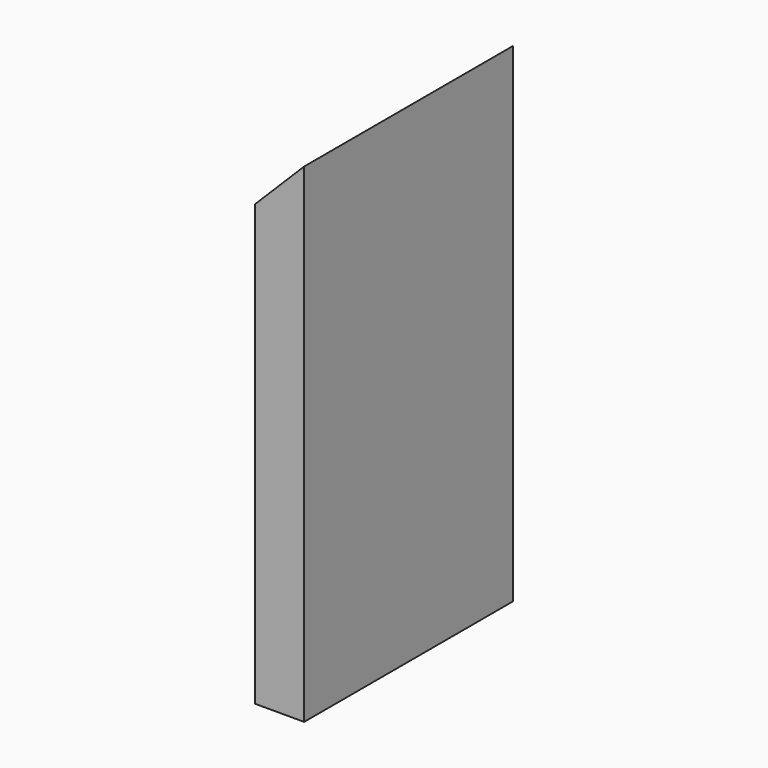
from build123d import *

# Parameters (mm, degrees)
F0_W     = 19.05
F0_H     = 101.6
F1_DEPTH = 190.5
F2_SIZE  = 19.04999


# Not quite as in the source:
# - a fillet or chamfer is up to 0.001 mm smaller than in the source, because OpenCascade refuses the exact size


with BuildPart() as f1:
    # F0 (on Top) → F1 (new body)
    with BuildSketch(Plane.XY):
        Rectangle(F0_W, F0_H)
    extrude(amount=F1_DEPTH)

    # F2 (size 19.05 in the source; OpenCascade refuses exactly that, so slightly less here)
    f2_edges = [f1.edges().sort_by_distance(p)[0] for p in [
        (-9.525, 0, 190.5),
    ]]
    chamfer(f2_edges, length=F2_SIZE)


solid = f1.part
